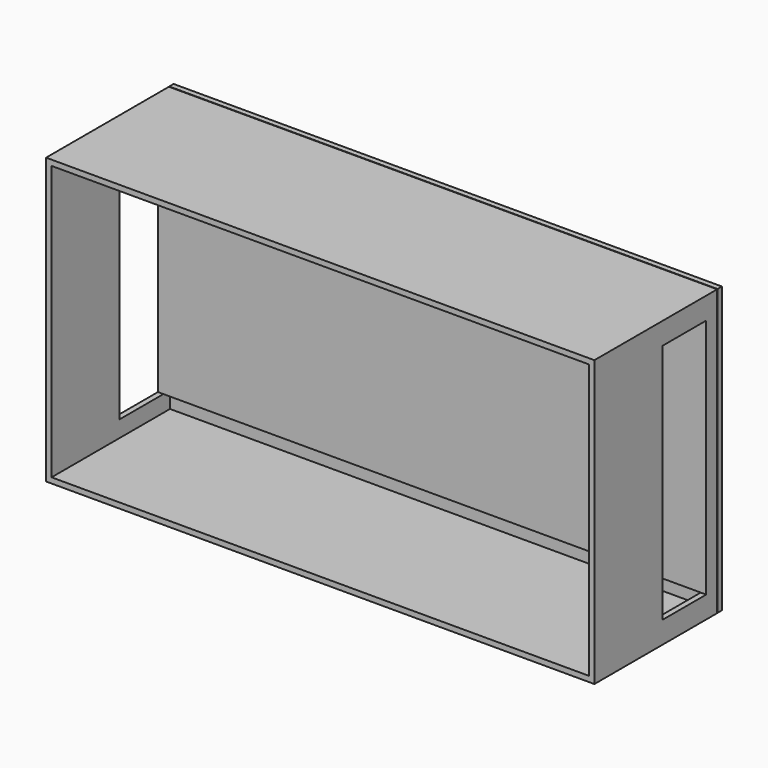
from build123d import *

# Parameters (mm, degrees)
F0_W     = 250
F0_H     = 130
F1_DEPTH = 2.5
F2_W     = 70
F2_H     = 130
F2_W_2   = 25
F2_H_2   = 110
F3_DEPTH = 125
F4_T     = 2.5


# Not quite as in the source:
# - a shell that OpenCascade refuses in one call is made with other operations: the cavity is built on its own and cut out


with BuildPart() as f1:
    # F0 (on Front) → F1 (new body)
    with BuildSketch(Plane.XZ):
        with Locations((0, 8.3088127774)):
            Rectangle(F0_W, F0_H)
    extrude(amount=F1_DEPTH)


with BuildPart() as f3:
    # F2 (on Right) → F3 (new body, symmetric)
    with BuildSketch(Plane.YZ):
        with Locations((-37.6844966412, 8.2720792294)):
            Rectangle(F2_W, F2_H)
        with Locations((-21.439858526, 8.2720792294)):
            Rectangle(F2_W_2, F2_H_2, mode=Mode.SUBTRACT)
    extrude(amount=F3_DEPTH, both=True)

    # F4: shell of thickness 2.5, made by hand


with BuildPart() as f4_core1:
    # F4_t2: copy of F3
    add(f3.part)

    # the walls: a layer under each face that stays
    f4_faces = [f4_core1.faces().sort_by_distance(p)[0] for p in [
        (0, -2.6844966412, 8.2720792294),
        (0, -37.6844966412, -56.7279207706),
        (125, -37.6844966412, 8.2720792294),
        (0, -8.939858526, 8.2720792294),
        (0, -37.6844966412, 73.2720792294),
        (-125, -37.6844966412, 8.2720792294),
    ]]
    thicken(f4_faces, amount=-F4_T, mode=Mode.SUBTRACT)


with BuildPart() as f3_1:
    add(f3.part)

    # what is left inside the walls is the cavity
    f4_cavity = [f4_core1.part.solids().sort_by_distance(p)[0] for p in [
        (-40.833333, -5.209497, 8.272079),
    ]]
    add(f4_cavity, mode=Mode.SUBTRACT)


solid = Compound([f1.part, f3_1.part])
